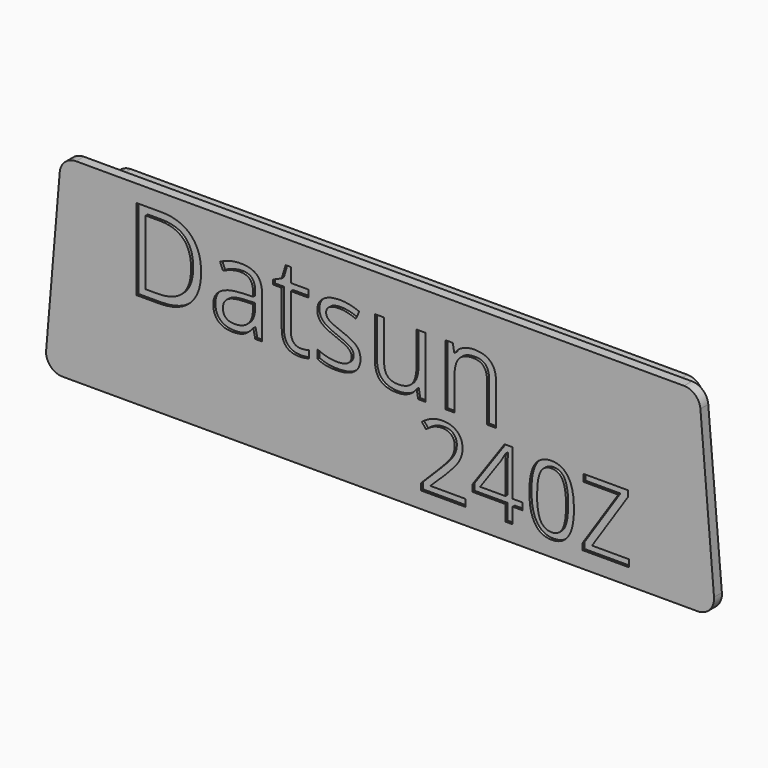
from build123d import *

# Parameters (mm, degrees)
F1_DEPTH       = 5
F3_DEPTH       = 3
F4_TEXT_SIZE   = 34.7553068423
F4_TEXT_SIZE_2 = 28.9070814486
F5_DEPTH       = 0.8


# Not quite as in the source:
# - Text() gives the source's letters only with a copy of the font that has no kerning and outlines rounded to 1/6400 em; it was checked with that copy


with BuildPart() as f1:
    # F0 (on Front) → F1 (new body)
    with BuildSketch(Plane.XZ):
        with BuildLine():
            Line((95.6309093535, 26.8134863051), (-74.3690906465, 26.8134863051))
            ThreePointArc((-74.3690906465, 26.8134863051), (-77.9046245524, 25.349020211), (-79.3690906465, 21.8134863051))
            Line((-79.3690906465, 21.8134863051), (-79.3690906465, -20.4865136949))
            ThreePointArc((-79.3690906465, -20.4865136949), (-77.9046245524, -24.0220476008), (-74.3690906465, -25.4865136949))
            Line((-74.3690906465, -25.4865136949), (95.6309093535, -25.4865136949))
            ThreePointArc((95.6309093535, -25.4865136949), (99.1664432594, -24.0220476008), (100.6309093535, -20.4865136949))
            Line((100.6309093535, -20.4865136949), (100.6309093535, 21.8134863051))
            ThreePointArc((100.6309093535, 21.8134863051), (99.1664432594, 25.349020211), (95.6309093535, 26.8134863051))
        make_face()
        with BuildLine():
            ThreePointArc((95.6309093535, 24.8134863051), (97.7522296971, 23.9348066487), (98.6309093535, 21.8134863051))
            Line((98.6309093535, 21.8134863051), (98.6309093535, -20.4865136949))
            ThreePointArc((98.6309093535, -20.4865136949), (97.7522296971, -22.6078340385), (95.6309093535, -23.4865136949))
            Line((95.6309093535, -23.4865136949), (-74.3690906465, -23.4865136949))
            ThreePointArc((-74.3690906465, -23.4865136949), (-76.4904109901, -22.6078340385), (-77.3690906465, -20.4865136949))
            Line((-77.3690906465, -20.4865136949), (-77.3690906465, 21.8134863051))
            ThreePointArc((-77.3690906465, 21.8134863051), (-76.4904109901, 23.9348066487), (-74.3690906465, 24.8134863051))
            Line((-74.3690906465, 24.8134863051), (95.6309093535, 24.8134863051))
        make_face(mode=Mode.SUBTRACT)
    extrude(amount=F1_DEPTH)

    # F2 (on face) → F3 (join)
    with BuildSketch(Plane.XZ.offset(5)):
        with BuildLine():
            Line((100.6309093535, 28.8134863051), (-79.3690906465, 28.8134863051))
            Line((-79.3690906465, 28.8134863051), (-84.7729338796, 28.8134863051))
            ThreePointArc((-84.7729338796, 28.8134863051), (-88.1566838323, 27.49455086), (-89.755254685, 24.2335808081))
            Line((-89.755254685, 24.2335808081), (-93.9120843646, -25.0664191919))
            ThreePointArc((-93.9120843646, -25.0664191919), (-92.6108281141, -28.8702636476), (-88.9297635592, -30.4865136949))
            Line((-88.9297635592, -30.4865136949), (-79.3690906465, -30.4865136949))
            Line((-79.3690906465, -30.4865136949), (100.6309093535, -30.4865136949))
            Line((100.6309093535, -30.4865136949), (105.1915822662, -30.4865136949))
            ThreePointArc((105.1915822662, -30.4865136949), (108.8726468211, -28.8702636476), (110.1739030716, -25.0664191919))
            Line((110.1739030716, -25.0664191919), (106.017073392, 24.2335808081))
            ThreePointArc((106.017073392, 24.2335808081), (104.4185025393, 27.49455086), (101.0347525866, 28.8134863051))
            Line((101.0347525866, 28.8134863051), (100.6309093535, 28.8134863051))
        make_face()
    extrude(amount=F3_DEPTH)

    # F4 (on face) → F5 (cut)
    with BuildSketch(Plane.XZ.offset(8)):
        with Locations((-69.7729338796, -1.2103346213)):
            Text('Datsun', F4_TEXT_SIZE, font='Open Sans', text_align=(TextAlign.LEFT, TextAlign.BOTTOM))
        with Locations((19.236810783, -25.4865136949)):
            Text('240Z', F4_TEXT_SIZE_2, font='Open Sans', text_align=(TextAlign.LEFT, TextAlign.BOTTOM))
    extrude(amount=-F5_DEPTH, mode=Mode.SUBTRACT)


solid = f1.part
